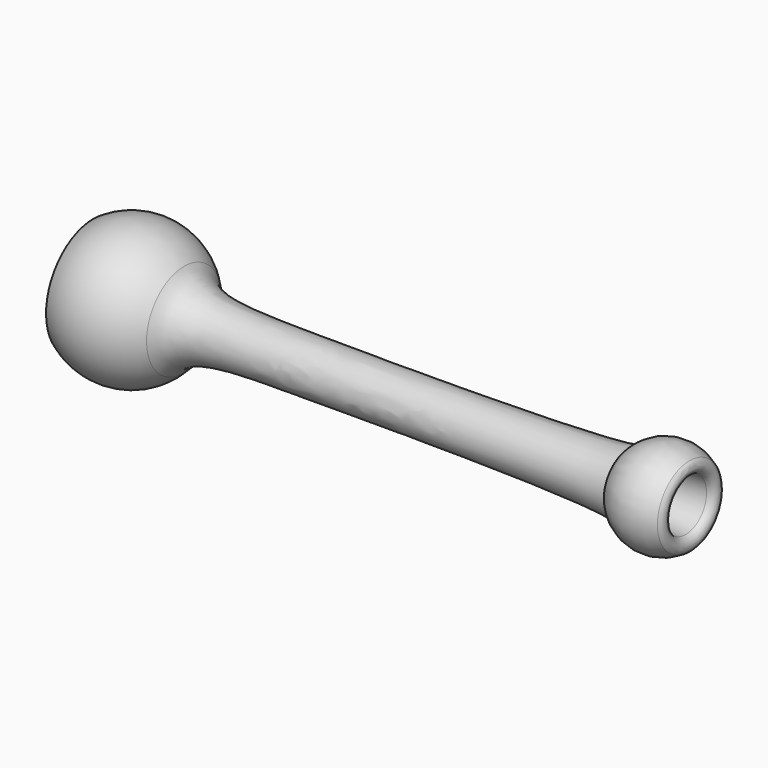
from build123d import *

# Parameters (mm, degrees)
F2_R = 2


# Not quite as in the source:
# - a fillet or chamfer that OpenCascade refuses, or shapes differently, is made with other operations: its cross-section is extruded or revolved along the edge and cut away or added


with BuildPart() as f1:
    # F0 (on Front) → F1 (revolve)
    with BuildSketch(Plane.XZ):
        with BuildLine():
            ThreePointArc((-7.0685046336, 10.3095219212), (4.6853520259, 11.5886788028), (12.2474487139, 2.5))
            Line((12.2474487139, 2.5), (74.2474487139, 2.5))
            Line((74.2474487139, 2.5), (149.7373398729, 7.1184875673))
            ThreePointArc((149.7373398729, 7.1184875673), (140.4668689382, 12.5188941968), (130.5825582503, 8.3467933662))
            add(Edge.make_bspline(
                [(13.7809895682, 12.3177978136), (17.1554645129, 6.7528548074), (43.3358067225, 6.5220205059), (122.1384170347, 6.3653155344), (130.5825582503, 8.3467933662)],
                knots=[0, 0, 0, 0, 0.3738465221, 1, 1, 1, 1], degree=3))
            ThreePointArc((13.7809895682, 12.3177978136), (2.4835532955, 18.3159979112), (-10.003236638, 15.5428141988))
            Line((-10.003236638, 15.5428141988), (-7.0685046336, 10.3095219212))
        make_face()
    revolve(axis=Axis((35, 0, 0), (1, 0, 0)))

    # F2
    f2_edges = [f1.edges().sort_by_distance(p)[0] for p in [
        (149.73734, 0, -7.118488),
        (-7.068505, 0, -10.309522),
        (12.247449, 0, -2.5),
    ]]
    fillet(f2_edges, radius=F2_R)

    # F3: fillet of radius 5 on 1 edges, made by hand

    # F3_s1 → F3_t2 (revolve, cut)
    with BuildSketch(Plane.XZ):
        with BuildLine():
            ThreePointArc((74.4000566425, 2.5089358376), (74.2473895925, 2.5019345041), (74.094579917, 2.4996))
            Line((74.094579917, 2.4996), (74.094579917, 1.99936))
            ThreePointArc((74.094579917, 1.99936), (74.1710143155, 1.99976), (74.2474487139, 1.99976))
            Line((74.2474487139, 1.99976), (74.2779963865, 2.0006935838))
            ThreePointArc((74.2779963865, 2.0006935838), (74.3542881375, 2.0053611293), (74.430604315, 2.0096294213))
            Line((74.430604315, 2.0096294213), (74.4000566425, 2.5089358376))
        make_face()
    revolve(axis=Axis((74.2474487139, 0, 0), (1, 0, 0)), mode=Mode.SUBTRACT)


solid = f1.part
